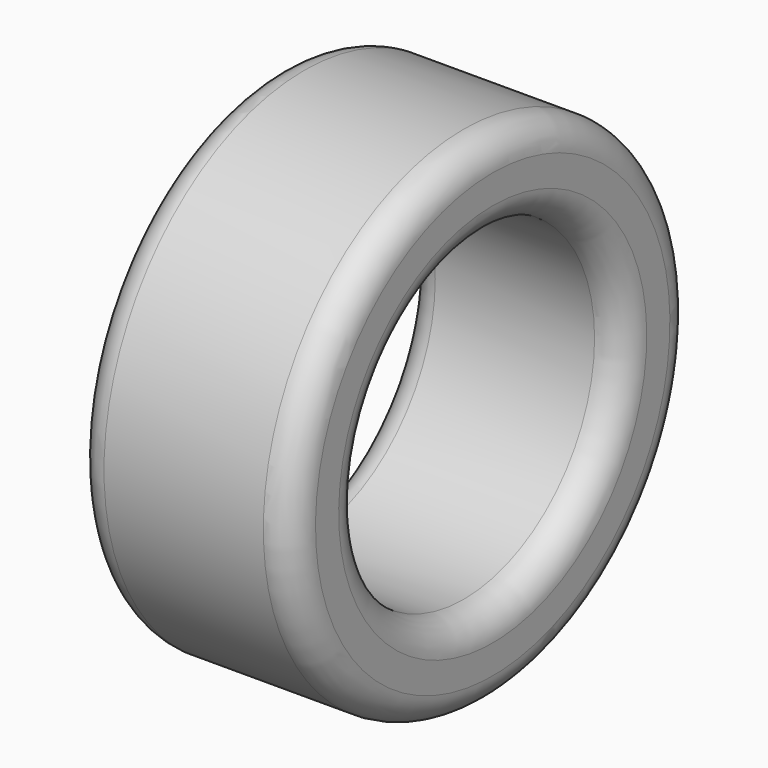
from build123d import *


# Not quite as in the source:
# - the program builds the solid bodies; features that only make, move or delete a surface that nothing else refers to are left out


with BuildPart() as f4:
    # F0 (on Front) → F4 (revolve)
    with BuildSketch(Plane.XZ):
        with BuildLine():
            ThreePointArc((-192.4457153976, -49.2647496334), (-177.5667398819, -85.1857741176), (-141.6457153976, -100.0647496334))
            Line((-141.6457153976, -100.0647496334), (137.7542846024, -100.0647496334))
            ThreePointArc((137.7542846024, -100.0647496334), (173.6753090867, -85.1857741176), (188.5542846024, -49.2647496334))
            Line((188.5542846024, -49.2647496334), (188.5542846024, 1.5352503666))
            ThreePointArc((188.5542846024, 1.5352503666), (173.6753090867, 37.4562748509), (137.7542846024, 52.3352503666))
            Line((137.7542846024, 52.3352503666), (-141.6457153976, 52.3352503666))
            ThreePointArc((-141.6457153976, 52.3352503666), (-177.5667398819, 37.4562748509), (-192.4457153976, 1.5352503666))
            Line((-192.4457153976, 1.5352503666), (-192.4457153976, -49.2647496334))
        make_face()
    revolve(axis=Axis((-11.0372006893, 0, -386.9243860245), (-1, 0, 0)))


solid = f4.part
